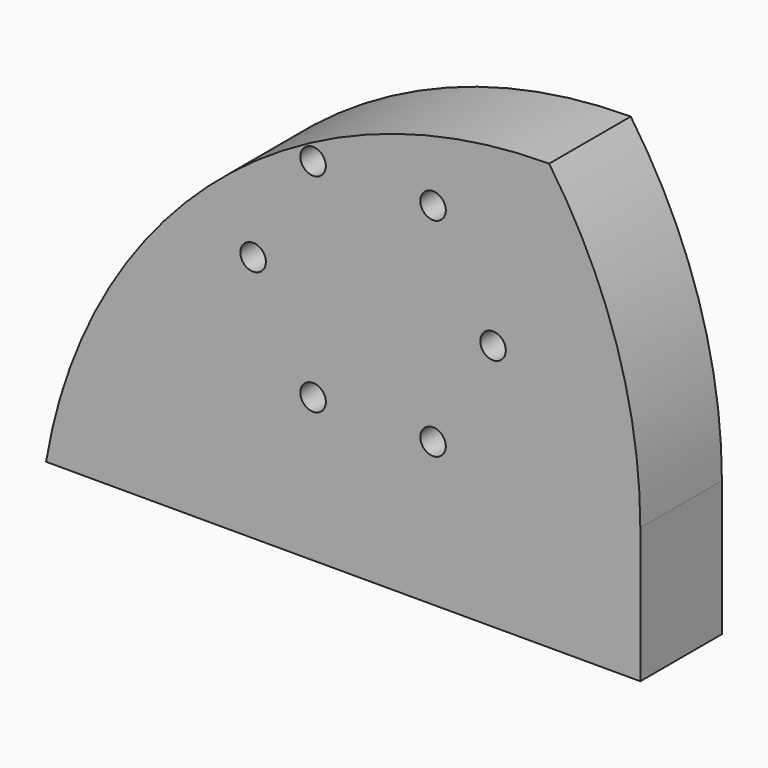
from build123d import *

# Parameters (mm, degrees)
F0_W        = 147.9716226459
F0_H        = 106.0937568545
F1_DEPTH    = 12.7
F2_T1_DEPTH = 651.7371495757
F3_T1_DEPTH = 387.7321882623
F5_D        = 6.35


# Not quite as in the source:
# - a fillet or chamfer that OpenCascade refuses, or shapes differently, is made with other operations: its cross-section is extruded or revolved along the edge and cut away or added


with BuildPart() as f1:
    # F0 (on Front) → F1 (new body, symmetric)
    with BuildSketch(Plane.XZ):
        with Locations((-0.1046992838, -8.5726827383)):
            Rectangle(F0_W, F0_H)
    extrude(amount=F1_DEPTH, both=True)

    # F2: fillet of radius 127 on 1 edges, made by hand

    # F2_s2 → F2_t1 (cut)
    with BuildSketch(Plane.XZ.offset(-325.8685747878)):
        with BuildLine():
            ThreePointArc((51.1769193084, 44.474195689), (-30.9020278112, 14.386766802), (-74.0905106068, -61.6195611656))
            Line((-74.0905106068, -61.6195611656), (-74.0905106068, 44.474195689))
            Line((-74.0905106068, 44.474195689), (51.1769193084, 44.474195689))
        make_face()
    extrude(amount=F2_T1_DEPTH, mode=Mode.SUBTRACT)

    # F3: fillet of radius 127 on 1 edges, made by hand

    # F3_s2 → F3_t1 (cut)
    with BuildSketch(Plane.XZ.offset(-193.8660941311)):
        with BuildLine():
            ThreePointArc((51.1769193084, 44.474195689), (68.0722163397, 9.9776966511), (73.8811120391, -27.9922419635))
            Line((73.8811120391, -27.9922419635), (73.8811120391, 44.474195689))
            Line((73.8811120391, 44.474195689), (51.1769193084, 44.474195689))
        make_face()
    extrude(amount=F3_T1_DEPTH, mode=Mode.SUBTRACT)

    # F5 (through all)
    with Locations(Plane.XZ.offset(12.7)):
        with Locations((-7.6034513134, -25.8695669472), (-22.5392527542, 0), (-7.6034513134, 25.8695669472), (22.2681515682, 25.8695669472), (37.203953009, 0), (22.2681515682, -25.8695669472)):
            Hole(F5_D / 2)


solid = f1.part
